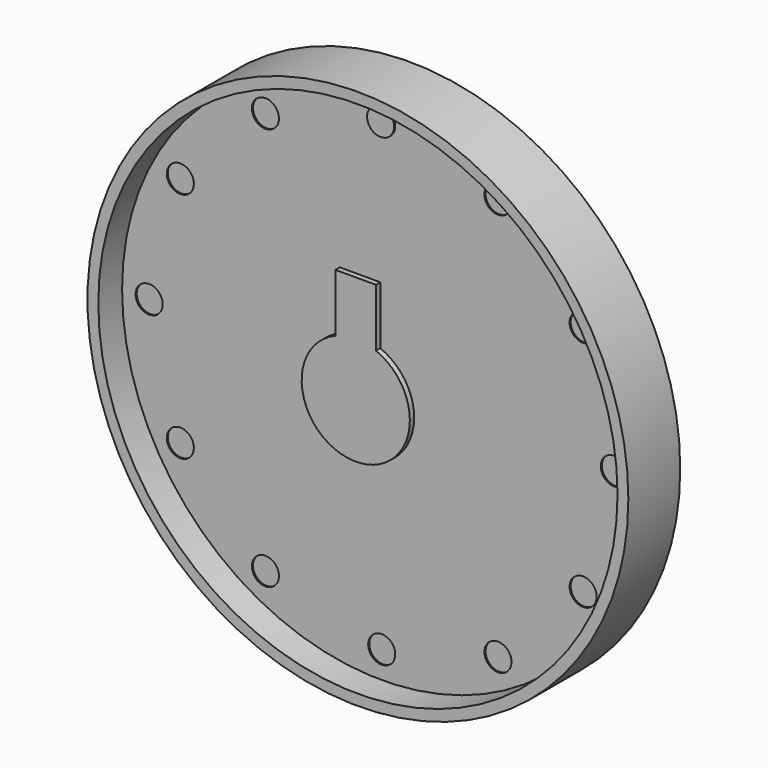
from build123d import *

# Parameters (mm, degrees)
F0_R      = 100
F1_DEPTH  = 24
F2_T      = -4
F3_R      = 5
F3_R_2    = 3
F4_DEPTH  = 6
F5_DEPTH  = 19
F6_DEPTH  = 8
F8_DEPTH  = 4
F10_DEPTH = 4
F11_R     = 5
F11_R_2   = 3
F12_DEPTH = 2
F13_R     = 98
F13_R_2   = 5
F14_DEPTH = 1
F16_R     = 5
F16_R_2   = 3
F17_DEPTH = 2
F18_R     = 5
F19_DEPTH = 0.5
F20_DEPTH = 1
F22_DEPTH = 2


with BuildPart() as f1:
    # F0 (on Front) → F1 (new body)
    with BuildSketch(Plane.XZ):
        Circle(F0_R)
    extrude(amount=F1_DEPTH)

    # F2
    f2_openings = [f1.faces().sort_by_distance(p)[0] for p in [
        (0, -24, 0),
    ]]
    offset(amount=F2_T, openings=f2_openings)

    # F3 (on Front) → F4 (join)
    with BuildSketch(Plane.XZ):
        with Locations((40, 0)):
            Circle(F3_R)
        with Locations((40, 0)):
            Circle(F3_R_2, mode=Mode.SUBTRACT)
        Circle(F3_R)
        Circle(F3_R_2, mode=Mode.SUBTRACT)
    extrude(amount=F4_DEPTH)


with BuildPart() as f5:
    # F5 (new): a face of the model
    f5_faces = [f1.part.faces().sort_by_distance(p)[0] for p in [
        (0, -4, 0),
    ]]
    extrude(f5_faces, amount=F5_DEPTH)

    # F7 (on face) → F8 (join)
    with BuildSketch(Plane.XZ.offset(6)):
        with BuildLine():
            ThreePointArc((9.2729637667, -1.3794085621), (9.3494561423, -0.6915886375), (9.375, 0))
            ThreePointArc((9.375, 0), (9.3494561423, 0.6915886375), (9.2729637667, 1.3794085621))
            ThreePointArc((9.2729637667, 1.3794085621), (8.9161548403, 2.8970343223), (8.3127812852, 4.3345463782))
            ThreePointArc((8.3127812852, 4.3345463782), (7.5845343223, 5.5104867402), (6.6911892658, 6.566476316))
            ThreePointArc((6.6911892658, 6.566476316), (5.5104867402, 7.5845343223), (4.1773988938, 8.3928519278))
            ThreePointArc((4.1773988938, 8.3928519278), (2.8970343223, 8.9161548403), (1.5536078905, 9.2453733036))
            ThreePointArc((1.5536078905, 9.2453733036), (0, 9.375), (-1.5536078905, 9.2453733036))
            ThreePointArc((-1.5536078905, 9.2453733036), (-2.8970343223, 8.9161548403), (-4.1773988938, 8.3928519278))
            ThreePointArc((-4.1773988938, 8.3928519278), (-5.5104867402, 7.5845343223), (-6.6911892658, 6.566476316))
            ThreePointArc((-6.6911892658, 6.566476316), (-7.5845343223, 5.5104867402), (-8.3127812852, 4.3345463782))
            ThreePointArc((-8.3127812852, 4.3345463782), (-8.9161548403, 2.8970343223), (-9.2729637667, 1.3794085621))
            ThreePointArc((-9.2729637667, 1.3794085621), (-9.375, 0), (-9.2729637667, -1.3794085621))
            ThreePointArc((-9.2729637667, -1.3794085621), (-8.9161548403, -2.8970343223), (-8.3127812852, -4.3345463782))
            ThreePointArc((-8.3127812852, -4.3345463782), (-7.5845343223, -5.5104867402), (-6.6911892658, -6.566476316))
            ThreePointArc((-6.6911892658, -6.566476316), (-5.5104867402, -7.5845343223), (-4.1773988938, -8.3928519278))
            ThreePointArc((-4.1773988938, -8.3928519278), (-2.8970343223, -8.9161548403), (-1.5536078905, -9.2453733036))
            ThreePointArc((-1.5536078905, -9.2453733036), (0, -9.375), (1.5536078905, -9.2453733036))
            ThreePointArc((1.5536078905, -9.2453733036), (2.8970343223, -8.9161548403), (4.1773988938, -8.3928519278))
            ThreePointArc((4.1773988938, -8.3928519278), (5.5104867402, -7.5845343223), (6.6911892658, -6.566476316))
            ThreePointArc((6.6911892658, -6.566476316), (7.5845343223, -5.5104867402), (8.3127812852, -4.3345463782))
            ThreePointArc((8.3127812852, -4.3345463782), (8.9161548403, -2.8970343223), (9.2729637667, -1.3794085621))
        make_face()
        with BuildLine():
            ThreePointArc((8.3127812852, 4.3345463782), (8.9161548403, 2.8970343223), (9.2729637667, 1.3794085621))
            Line((9.2729637667, 1.3794085621), (11.1823199426, 2.3946312492))
            Line((11.1823199426, 2.3946312492), (10.8182678729, 3.515068311))
            Line((10.8182678729, 3.515068311), (10.4542158031, 4.6355053728))
            Line((10.4542158031, 4.6355053728), (8.3127812852, 4.3345463782))
        make_face()
        with BuildLine():
            Line((11.1823199426, -2.3946312492), (9.2729637667, -1.3794085621))
            ThreePointArc((9.2729637667, -1.3794085621), (8.9161548403, -2.8970343223), (8.3127812852, -4.3345463782))
            Line((8.3127812852, -4.3345463782), (10.4542158031, -4.6355053728))
            Line((10.4542158031, -4.6355053728), (10.8182678729, -3.515068311))
            Line((10.8182678729, -3.515068311), (11.1823199426, -2.3946312492))
        make_face()
        with BuildLine():
            ThreePointArc((4.1773988938, 8.3928519278), (5.5104867402, 7.5845343223), (6.6911892658, 6.566476316))
            Line((6.6911892658, 6.566476316), (7.6391579371, 8.5101001246))
            Line((7.6391579371, 8.5101001246), (6.6860572448, 9.202568311))
            Line((6.6860572448, 9.202568311), (5.7329565525, 9.8950364974))
            Line((5.7329565525, 9.8950364974), (4.1773988938, 8.3928519278))
        make_face()
        with BuildLine():
            Line((7.6391579371, -8.5101001246), (6.6911892658, -6.566476316))
            ThreePointArc((6.6911892658, -6.566476316), (5.5104867402, -7.5845343223), (4.1773988938, -8.3928519278))
            Line((4.1773988938, -8.3928519278), (5.7329565525, -9.8950364974))
            Line((5.7329565525, -9.8950364974), (6.6860572448, -9.202568311))
            Line((6.6860572448, -9.202568311), (7.6391579371, -8.5101001246))
        make_face()
        with BuildLine():
            ThreePointArc((-1.5536078905, 9.2453733036), (0, 9.375), (1.5536078905, 9.2453733036))
            Line((1.5536078905, 9.2453733036), (1.1780972451, 11.375))
            Line((1.1780972451, 11.375), (0, 11.375))
            Line((0, 11.375), (-1.1780972451, 11.375))
            Line((-1.1780972451, 11.375), (-1.5536078905, 9.2453733036))
        make_face()
        with BuildLine():
            Line((1.1780972451, -11.375), (1.5536078905, -9.2453733036))
            ThreePointArc((1.5536078905, -9.2453733036), (0, -9.375), (-1.5536078905, -9.2453733036))
            Line((-1.5536078905, -9.2453733036), (-1.1780972451, -11.375))
            Line((-1.1780972451, -11.375), (0, -11.375))
            Line((0, -11.375), (1.1780972451, -11.375))
        make_face()
        with BuildLine():
            ThreePointArc((-6.6911892658, 6.566476316), (-5.5104867402, 7.5845343223), (-4.1773988938, 8.3928519278))
            Line((-4.1773988938, 8.3928519278), (-5.7329565525, 9.8950364974))
            Line((-5.7329565525, 9.8950364974), (-6.6860572448, 9.202568311))
            Line((-6.6860572448, 9.202568311), (-7.6391579371, 8.5101001246))
            Line((-7.6391579371, 8.5101001246), (-6.6911892658, 6.566476316))
        make_face()
        with BuildLine():
            Line((-5.7329565525, -9.8950364974), (-4.1773988938, -8.3928519278))
            ThreePointArc((-4.1773988938, -8.3928519278), (-5.5104867402, -7.5845343223), (-6.6911892658, -6.566476316))
            Line((-6.6911892658, -6.566476316), (-7.6391579371, -8.5101001246))
            Line((-7.6391579371, -8.5101001246), (-6.6860572448, -9.202568311))
            Line((-6.6860572448, -9.202568311), (-5.7329565525, -9.8950364974))
        make_face()
        with BuildLine():
            ThreePointArc((-9.2729637667, 1.3794085621), (-8.9161548403, 2.8970343223), (-8.3127812852, 4.3345463782))
            Line((-8.3127812852, 4.3345463782), (-10.4542158031, 4.6355053728))
            Line((-10.4542158031, 4.6355053728), (-10.8182678729, 3.515068311))
            Line((-10.8182678729, 3.515068311), (-11.1823199426, 2.3946312492))
            Line((-11.1823199426, 2.3946312492), (-9.2729637667, 1.3794085621))
        make_face()
        with BuildLine():
            Line((-10.4542158031, -4.6355053728), (-8.3127812852, -4.3345463782))
            ThreePointArc((-8.3127812852, -4.3345463782), (-8.9161548403, -2.8970343223), (-9.2729637667, -1.3794085621))
            Line((-9.2729637667, -1.3794085621), (-11.1823199426, -2.3946312492))
            Line((-11.1823199426, -2.3946312492), (-10.8182678729, -3.515068311))
            Line((-10.8182678729, -3.515068311), (-10.4542158031, -4.6355053728))
        make_face()
    extrude(amount=F8_DEPTH)

    # F21 (on face) → F22 (join)
    with BuildSketch(Plane.XZ.offset(23)):
        with BuildLine():
            ThreePointArc((-7.5, 18.5404962177), (-11.1803398875, -16.5831239518), (20, 0))
            ThreePointArc((20, 0), (16.5831239518, 11.1803398875), (7.5, 18.5404962177))
            ThreePointArc((7.5, 18.5404962177), (0, 20), (-7.5, 18.5404962177))
        make_face()
        with BuildLine():
            ThreePointArc((-7.5, 18.5404962177), (0, 20), (7.5, 18.5404962177))
            Line((7.5, 18.5404962177), (7.5, 40))
            Line((7.5, 40), (0, 40))
            Line((0, 40), (-7.5, 40))
            Line((-7.5, 40), (-7.5, 18.5404962177))
        make_face()
    extrude(amount=F22_DEPTH)


with BuildPart() as f6:
    # F6 (new): a face of the model
    f6_faces = [f1.part.faces().sort_by_distance(p)[0] for p in [
        (40, -4, 0),
    ]]
    extrude(f6_faces, amount=F6_DEPTH)

    # F9 (on face) → F10 (join)
    with BuildSketch(Plane.XZ.offset(6)):
        with BuildLine():
            ThreePointArc((68.0829066802, -1.5381733945), (68.1144747006, -0.7693746225), (68.125, 0))
            ThreePointArc((68.125, 0), (68.1144747006, 0.7693746225), (68.0829066802, 1.5381733945))
            ThreePointArc((68.0829066802, 1.5381733945), (67.9709283072, 2.9398630294), (67.7890320221, 4.3342039956))
            ThreePointArc((67.7890320221, 4.3342039956), (67.5104012706, 5.8475163042), (67.1494235596, 7.3433252263))
            ThreePointArc((67.1494235596, 7.3433252263), (66.7484645208, 8.6911029668), (66.280643318, 10.0171558733))
            ThreePointArc((66.280643318, 10.0171558733), (65.6934659962, 11.4394680865), (65.0293803521, 12.8275385085))
            ThreePointArc((65.0293803521, 12.8275385085), (64.3569644814, 14.0625), (63.6236643925, 15.2623099717))
            ThreePointArc((63.6236643925, 15.2623099717), (62.7536029668, 16.5314602207), (61.815433119, 17.7511268046))
            ThreePointArc((61.815433119, 17.7511268046), (60.9009482166, 18.8192983038), (59.934217974, 19.8404278876))
            ThreePointArc((59.934217974, 19.8404278876), (58.8192983038, 20.9009482166), (57.6480467764, 21.8989056799))
            ThreePointArc((57.6480467764, 21.8989056799), (56.5314602207, 22.7536029668), (55.3735505752, 23.5514238999))
            ThreePointArc((55.3735505752, 23.5514238999), (54.0625, 24.3569644814), (52.709356105, 25.0895972944))
            ThreePointArc((52.709356105, 25.0895972944), (51.4394680865, 25.6934659962), (50.1409852457, 26.2331096755))
            ThreePointArc((50.1409852457, 26.2331096755), (48.6911029668, 26.7484645208), (47.2152055856, 27.1837531139))
            ThreePointArc((47.2152055856, 27.1837531139), (45.8475163042, 27.5104012706), (44.4652101991, 27.7682826779))
            ThreePointArc((44.4652101991, 27.7682826779), (42.9398630294, 27.9709283072), (41.4057159597, 28.0898484802))
            ThreePointArc((41.4057159597, 28.0898484802), (40, 28.125), (38.5942840403, 28.0898484802))
            ThreePointArc((38.5942840403, 28.0898484802), (37.0601369706, 27.9709283072), (35.5347898009, 27.7682826779))
            ThreePointArc((35.5347898009, 27.7682826779), (34.1524836958, 27.5104012706), (32.7847944144, 27.1837531139))
            ThreePointArc((32.7847944144, 27.1837531139), (31.3088970332, 26.7484645208), (29.8590147543, 26.2331096755))
            ThreePointArc((29.8590147543, 26.2331096755), (28.5605319135, 25.6934659962), (27.290643895, 25.0895972944))
            ThreePointArc((27.290643895, 25.0895972944), (25.9375, 24.3569644814), (24.6264494248, 23.5514238999))
            ThreePointArc((24.6264494248, 23.5514238999), (23.4685397793, 22.7536029668), (22.3519532236, 21.8989056799))
            ThreePointArc((22.3519532236, 21.8989056799), (21.1807016962, 20.9009482166), (20.065782026, 19.8404278876))
            ThreePointArc((20.065782026, 19.8404278876), (19.0990517834, 18.8192983038), (18.184566881, 17.7511268046))
            ThreePointArc((18.184566881, 17.7511268046), (17.2463970332, 16.5314602207), (16.3763356075, 15.2623099717))
            ThreePointArc((16.3763356075, 15.2623099717), (15.6430355186, 14.0625), (14.9706196479, 12.8275385085))
            ThreePointArc((14.9706196479, 12.8275385085), (14.3065340038, 11.4394680865), (13.719356682, 10.0171558733))
            ThreePointArc((13.719356682, 10.0171558733), (13.2515354792, 8.6911029668), (12.8505764404, 7.3433252263))
            ThreePointArc((12.8505764404, 7.3433252263), (12.4895987294, 5.8475163042), (12.2109679779, 4.3342039956))
            ThreePointArc((12.2109679779, 4.3342039956), (12.0290716928, 2.9398630294), (11.9170933198, 1.5381733945))
            ThreePointArc((11.9170933198, 1.5381733945), (11.875, 0), (11.9170933198, -1.5381733945))
            ThreePointArc((11.9170933198, -1.5381733945), (12.0290716928, -2.9398630294), (12.2109679779, -4.3342039956))
            ThreePointArc((12.2109679779, -4.3342039956), (12.4895987294, -5.8475163042), (12.8505764404, -7.3433252263))
            ThreePointArc((12.8505764404, -7.3433252263), (13.2515354792, -8.6911029668), (13.719356682, -10.0171558733))
            ThreePointArc((13.719356682, -10.0171558733), (14.3065340038, -11.4394680865), (14.9706196479, -12.8275385085))
            ThreePointArc((14.9706196479, -12.8275385085), (15.6430355186, -14.0625), (16.3763356075, -15.2623099717))
            ThreePointArc((16.3763356075, -15.2623099717), (17.2463970332, -16.5314602207), (18.184566881, -17.7511268046))
            ThreePointArc((18.184566881, -17.7511268046), (19.0990517834, -18.8192983038), (20.065782026, -19.8404278876))
            ThreePointArc((20.065782026, -19.8404278876), (21.1807016962, -20.9009482166), (22.3519532236, -21.8989056799))
            ThreePointArc((22.3519532236, -21.8989056799), (23.4685397793, -22.7536029668), (24.6264494248, -23.5514238999))
            ThreePointArc((24.6264494248, -23.5514238999), (25.9375, -24.3569644814), (27.290643895, -25.0895972944))
            ThreePointArc((27.290643895, -25.0895972944), (28.5605319135, -25.6934659962), (29.8590147543, -26.2331096755))
            ThreePointArc((29.8590147543, -26.2331096755), (31.3088970332, -26.7484645208), (32.7847944144, -27.1837531139))
            ThreePointArc((32.7847944144, -27.1837531139), (34.1524836958, -27.5104012706), (35.5347898009, -27.7682826779))
            ThreePointArc((35.5347898009, -27.7682826779), (37.0601369706, -27.9709283072), (38.5942840403, -28.0898484802))
            ThreePointArc((38.5942840403, -28.0898484802), (40, -28.125), (41.4057159597, -28.0898484802))
            ThreePointArc((41.4057159597, -28.0898484802), (42.9398630294, -27.9709283072), (44.4652101991, -27.7682826779))
            ThreePointArc((44.4652101991, -27.7682826779), (45.8475163042, -27.5104012706), (47.2152055856, -27.1837531139))
            ThreePointArc((47.2152055856, -27.1837531139), (48.6911029668, -26.7484645208), (50.1409852457, -26.2331096755))
            ThreePointArc((50.1409852457, -26.2331096755), (51.4394680865, -25.6934659962), (52.709356105, -25.0895972944))
            ThreePointArc((52.709356105, -25.0895972944), (54.0625, -24.3569644814), (55.3735505752, -23.5514238999))
            ThreePointArc((55.3735505752, -23.5514238999), (56.5314602207, -22.7536029668), (57.6480467764, -21.8989056799))
            ThreePointArc((57.6480467764, -21.8989056799), (58.8192983038, -20.9009482166), (59.934217974, -19.8404278876))
            ThreePointArc((59.934217974, -19.8404278876), (60.9009482166, -18.8192983038), (61.815433119, -17.7511268046))
            ThreePointArc((61.815433119, -17.7511268046), (62.7536029668, -16.5314602207), (63.6236643925, -15.2623099717))
            ThreePointArc((63.6236643925, -15.2623099717), (64.3569644814, -14.0625), (65.0293803521, -12.8275385085))
            ThreePointArc((65.0293803521, -12.8275385085), (65.6934659962, -11.4394680865), (66.280643318, -10.0171558733))
            ThreePointArc((66.280643318, -10.0171558733), (66.7484645208, -8.6911029668), (67.1494235596, -7.3433252263))
            ThreePointArc((67.1494235596, -7.3433252263), (67.5104012706, -5.8475163042), (67.7890320221, -4.3342039956))
            ThreePointArc((67.7890320221, -4.3342039956), (67.9709283072, -2.9398630294), (68.0829066802, -1.5381733945))
        make_face()
        with BuildLine():
            ThreePointArc((68.0829066802, 1.5381733945), (68.1144747006, 0.7693746225), (68.125, 0))
            ThreePointArc((68.125, 0), (68.1144747006, -0.7693746225), (68.0829066802, -1.5381733945))
            Line((68.0829066802, -1.5381733945), (70.125, -1.1780972451))
            Line((70.125, -1.1780972451), (70.125, 0))
            Line((70.125, 0), (70.125, 1.1780972451))
            Line((70.125, 1.1780972451), (68.0829066802, 1.5381733945))
        make_face()
        with BuildLine():
            ThreePointArc((67.1494235596, 7.3433252263), (67.5104012706, 5.8475163042), (67.7890320221, 4.3342039956))
            Line((67.7890320221, 4.3342039956), (69.7116366623, 5.1109866922))
            Line((69.7116366623, 5.1109866922), (69.4666964721, 6.2633396859))
            Line((69.4666964721, 6.2633396859), (69.2217562819, 7.4156926796))
            Line((69.2217562819, 7.4156926796), (67.1494235596, 7.3433252263))
        make_face()
        with BuildLine():
            Line((69.7116366623, -5.1109866922), (67.7890320221, -4.3342039956))
            ThreePointArc((67.7890320221, -4.3342039956), (67.5104012706, -5.8475163042), (67.1494235596, -7.3433252263))
            Line((67.1494235596, -7.3433252263), (69.2217562819, -7.4156926796))
            Line((69.2217562819, -7.4156926796), (69.4666964721, -6.2633396859))
            Line((69.4666964721, -6.2633396859), (69.7116366623, -5.1109866922))
        make_face()
        with BuildLine():
            ThreePointArc((65.0293803521, 12.8275385085), (65.6934659962, 11.4394680865), (66.280643318, 10.0171558733))
            Line((66.280643318, 10.0171558733), (67.9997322302, 11.1766959857))
            Line((67.9997322302, 11.1766959857), (67.5205569115, 12.2529413727))
            Line((67.5205569115, 12.2529413727), (67.0413815928, 13.3291867596))
            Line((67.0413815928, 13.3291867596), (65.0293803521, 12.8275385085))
        make_face()
        with BuildLine():
            Line((67.9997322302, -11.1766959857), (66.280643318, -10.0171558733))
            ThreePointArc((66.280643318, -10.0171558733), (65.6934659962, -11.4394680865), (65.0293803521, -12.8275385085))
            Line((65.0293803521, -12.8275385085), (67.0413815928, -13.3291867596))
            Line((67.0413815928, -13.3291867596), (67.5205569115, -12.2529413727))
            Line((67.5205569115, -12.2529413727), (67.9997322302, -11.1766959857))
        make_face()
        with BuildLine():
            ThreePointArc((61.815433119, 17.7511268046), (62.7536029668, 16.5314602207), (63.6236643925, 15.2623099717))
            Line((63.6236643925, 15.2623099717), (65.064105142, 16.753930033))
            Line((65.064105142, 16.753930033), (64.3716369555, 17.7070307253))
            Line((64.3716369555, 17.7070307253), (63.6791687691, 18.6601314176))
            Line((63.6791687691, 18.6601314176), (61.815433119, 17.7511268046))
        make_face()
        with BuildLine():
            Line((65.064105142, -16.753930033), (63.6236643925, -15.2623099717))
            ThreePointArc((63.6236643925, -15.2623099717), (62.7536029668, -16.5314602207), (61.815433119, -17.7511268046))
            Line((61.815433119, -17.7511268046), (63.6791687691, -18.6601314176))
            Line((63.6791687691, -18.6601314176), (64.3716369555, -17.7070307253))
            Line((64.3716369555, -17.7070307253), (65.064105142, -16.753930033))
        make_face()
        with BuildLine():
            ThreePointArc((57.6480467764, 21.8989056799), (58.8192983038, 20.9009482166), (59.934217974, 19.8404278876))
            Line((59.934217974, 19.8404278876), (61.0330563882, 21.5989369435))
            Line((61.0330563882, 21.5989369435), (60.1575595166, 22.3872378675))
            Line((60.1575595166, 22.3872378675), (59.282062645, 23.1755387915))
            Line((59.282062645, 23.1755387915), (57.6480467764, 21.8989056799))
        make_face()
        with BuildLine():
            Line((61.0330563882, -21.5989369435), (59.934217974, -19.8404278876))
            ThreePointArc((59.934217974, -19.8404278876), (58.8192983038, -20.9009482166), (57.6480467764, -21.8989056799))
            Line((57.6480467764, -21.8989056799), (59.282062645, -23.1755387915))
            Line((59.282062645, -23.1755387915), (60.1575595166, -22.3872378675))
            Line((60.1575595166, -22.3872378675), (61.0330563882, -21.5989369435))
        make_face()
        with BuildLine():
            ThreePointArc((52.709356105, 25.0895972944), (54.0625, 24.3569644814), (55.3735505752, 23.5514238999))
            Line((55.3735505752, 23.5514238999), (56.0827621424, 25.4999666665))
            Line((56.0827621424, 25.4999666665), (55.0625, 26.089015289))
            Line((55.0625, 26.089015289), (54.0422378576, 26.6780639116))
            Line((54.0422378576, 26.6780639116), (52.709356105, 25.0895972944))
        make_face()
        with BuildLine():
            Line((56.0827621424, -25.4999666665), (55.3735505752, -23.5514238999))
            ThreePointArc((55.3735505752, -23.5514238999), (54.0625, -24.3569644814), (52.709356105, -25.0895972944))
            Line((52.709356105, -25.0895972944), (54.0422378576, -26.6780639116))
            Line((54.0422378576, -26.6780639116), (55.0625, -26.089015289))
            Line((55.0625, -26.089015289), (56.0827621424, -25.4999666665))
        make_face()
        with BuildLine():
            ThreePointArc((47.2152055856, 27.1837531139), (48.6911029668, 26.7484645208), (50.1409852457, 26.2331096755))
            Line((50.1409852457, 26.2331096755), (50.4295740173, 28.2865254836))
            Line((50.4295740173, 28.2865254836), (49.3091369555, 28.6505775534))
            Line((49.3091369555, 28.6505775534), (48.1886998938, 29.0146296232))
            Line((48.1886998938, 29.0146296232), (47.2152055856, 27.1837531139))
        make_face()
        with BuildLine():
            Line((50.4295740173, -28.2865254836), (50.1409852457, -26.2331096755))
            ThreePointArc((50.1409852457, -26.2331096755), (48.6911029668, -26.7484645208), (47.2152055856, -27.1837531139))
            Line((47.2152055856, -27.1837531139), (48.1886998938, -29.0146296232))
            Line((48.1886998938, -29.0146296232), (49.3091369555, -28.6505775534))
            Line((49.3091369555, -28.6505775534), (50.4295740173, -28.2865254836))
        make_face()
        with BuildLine():
            ThreePointArc((41.4057159597, 28.0898484802), (42.9398630294, 27.9709283072), (44.4652101991, 27.7682826779))
            Line((44.4652101991, 27.7682826779), (44.3205634611, 29.8368274034))
            Line((44.3205634611, 29.8368274034), (43.1489199559, 29.959972098))
            Line((43.1489199559, 29.959972098), (41.9772764508, 30.0831167926))
            Line((41.9772764508, 30.0831167926), (41.4057159597, 28.0898484802))
        make_face()
        with BuildLine():
            Line((44.3205634611, -29.8368274034), (44.4652101991, -27.7682826779))
            ThreePointArc((44.4652101991, -27.7682826779), (42.9398630294, -27.9709283072), (41.4057159597, -28.0898484802))
            Line((41.4057159597, -28.0898484802), (41.9772764508, -30.0831167926))
            Line((41.9772764508, -30.0831167926), (43.1489199559, -29.959972098))
            Line((43.1489199559, -29.959972098), (44.3205634611, -29.8368274034))
        make_face()
        with BuildLine():
            ThreePointArc((35.5347898009, 27.7682826779), (37.0601369706, 27.9709283072), (38.5942840403, 28.0898484802))
            Line((38.5942840403, 28.0898484802), (38.0227235492, 30.0831167926))
            Line((38.0227235492, 30.0831167926), (36.8510800441, 29.959972098))
            Line((36.8510800441, 29.959972098), (35.6794365389, 29.8368274034))
            Line((35.6794365389, 29.8368274034), (35.5347898009, 27.7682826779))
        make_face()
        with BuildLine():
            Line((38.0227235492, -30.0831167926), (38.5942840403, -28.0898484802))
            ThreePointArc((38.5942840403, -28.0898484802), (37.0601369706, -27.9709283072), (35.5347898009, -27.7682826779))
            Line((35.5347898009, -27.7682826779), (35.6794365389, -29.8368274034))
            Line((35.6794365389, -29.8368274034), (36.8510800441, -29.959972098))
            Line((36.8510800441, -29.959972098), (38.0227235492, -30.0831167926))
        make_face()
        with BuildLine():
            ThreePointArc((29.8590147543, 26.2331096755), (31.3088970332, 26.7484645208), (32.7847944144, 27.1837531139))
            Line((32.7847944144, 27.1837531139), (31.8113001062, 29.0146296232))
            Line((31.8113001062, 29.0146296232), (30.6908630445, 28.6505775534))
            Line((30.6908630445, 28.6505775534), (29.5704259827, 28.2865254836))
            Line((29.5704259827, 28.2865254836), (29.8590147543, 26.2331096755))
        make_face()
        with BuildLine():
            Line((31.8113001062, -29.0146296232), (32.7847944144, -27.1837531139))
            ThreePointArc((32.7847944144, -27.1837531139), (31.3088970332, -26.7484645208), (29.8590147543, -26.2331096755))
            Line((29.8590147543, -26.2331096755), (29.5704259827, -28.2865254836))
            Line((29.5704259827, -28.2865254836), (30.6908630445, -28.6505775534))
            Line((30.6908630445, -28.6505775534), (31.8113001062, -29.0146296232))
        make_face()
        with BuildLine():
            ThreePointArc((24.6264494248, 23.5514238999), (25.9375, 24.3569644814), (27.290643895, 25.0895972944))
            Line((27.290643895, 25.0895972944), (25.9577621424, 26.6780639116))
            Line((25.9577621424, 26.6780639116), (24.9375, 26.089015289))
            Line((24.9375, 26.089015289), (23.9172378576, 25.4999666665))
            Line((23.9172378576, 25.4999666665), (24.6264494248, 23.5514238999))
        make_face()
        with BuildLine():
            Line((25.9577621424, -26.6780639116), (27.290643895, -25.0895972944))
            ThreePointArc((27.290643895, -25.0895972944), (25.9375, -24.3569644814), (24.6264494248, -23.5514238999))
            Line((24.6264494248, -23.5514238999), (23.9172378576, -25.4999666665))
            Line((23.9172378576, -25.4999666665), (24.9375, -26.089015289))
            Line((24.9375, -26.089015289), (25.9577621424, -26.6780639116))
        make_face()
        with BuildLine():
            ThreePointArc((20.065782026, 19.8404278876), (21.1807016962, 20.9009482166), (22.3519532236, 21.8989056799))
            Line((22.3519532236, 21.8989056799), (20.717937355, 23.1755387915))
            Line((20.717937355, 23.1755387915), (19.8424404834, 22.3872378675))
            Line((19.8424404834, 22.3872378675), (18.9669436118, 21.5989369435))
            Line((18.9669436118, 21.5989369435), (20.065782026, 19.8404278876))
        make_face()
        with BuildLine():
            Line((20.717937355, -23.1755387915), (22.3519532236, -21.8989056799))
            ThreePointArc((22.3519532236, -21.8989056799), (21.1807016962, -20.9009482166), (20.065782026, -19.8404278876))
            Line((20.065782026, -19.8404278876), (18.9669436118, -21.5989369435))
            Line((18.9669436118, -21.5989369435), (19.8424404834, -22.3872378675))
            Line((19.8424404834, -22.3872378675), (20.717937355, -23.1755387915))
        make_face()
        with BuildLine():
            ThreePointArc((16.3763356075, 15.2623099717), (17.2463970332, 16.5314602207), (18.184566881, 17.7511268046))
            Line((18.184566881, 17.7511268046), (16.3208312309, 18.6601314176))
            Line((16.3208312309, 18.6601314176), (15.6283630445, 17.7070307253))
            Line((15.6283630445, 17.7070307253), (14.935894858, 16.753930033))
            Line((14.935894858, 16.753930033), (16.3763356075, 15.2623099717))
        make_face()
        with BuildLine():
            Line((16.3208312309, -18.6601314176), (18.184566881, -17.7511268046))
            ThreePointArc((18.184566881, -17.7511268046), (17.2463970332, -16.5314602207), (16.3763356075, -15.2623099717))
            Line((16.3763356075, -15.2623099717), (14.935894858, -16.753930033))
            Line((14.935894858, -16.753930033), (15.6283630445, -17.7070307253))
            Line((15.6283630445, -17.7070307253), (16.3208312309, -18.6601314176))
        make_face()
        with BuildLine():
            ThreePointArc((13.719356682, 10.0171558733), (14.3065340038, 11.4394680865), (14.9706196479, 12.8275385085))
            Line((14.9706196479, 12.8275385085), (12.9586184072, 13.3291867596))
            Line((12.9586184072, 13.3291867596), (12.4794430885, 12.2529413727))
            Line((12.4794430885, 12.2529413727), (12.0002677698, 11.1766959857))
            Line((12.0002677698, 11.1766959857), (13.719356682, 10.0171558733))
        make_face()
        with BuildLine():
            Line((12.9586184072, -13.3291867596), (14.9706196479, -12.8275385085))
            ThreePointArc((14.9706196479, -12.8275385085), (14.3065340038, -11.4394680865), (13.719356682, -10.0171558733))
            Line((13.719356682, -10.0171558733), (12.0002677698, -11.1766959857))
            Line((12.0002677698, -11.1766959857), (12.4794430885, -12.2529413727))
            Line((12.4794430885, -12.2529413727), (12.9586184072, -13.3291867596))
        make_face()
        with BuildLine():
            ThreePointArc((12.2109679779, 4.3342039956), (12.4895987294, 5.8475163042), (12.8505764404, 7.3433252263))
            Line((12.8505764404, 7.3433252263), (10.7782437181, 7.4156926796))
            Line((10.7782437181, 7.4156926796), (10.5333035279, 6.2633396859))
            Line((10.5333035279, 6.2633396859), (10.2883633377, 5.1109866922))
            Line((10.2883633377, 5.1109866922), (12.2109679779, 4.3342039956))
        make_face()
        with BuildLine():
            Line((10.7782437181, -7.4156926796), (12.8505764404, -7.3433252263))
            ThreePointArc((12.8505764404, -7.3433252263), (12.4895987294, -5.8475163042), (12.2109679779, -4.3342039956))
            Line((12.2109679779, -4.3342039956), (10.2883633377, -5.1109866922))
            Line((10.2883633377, -5.1109866922), (10.5333035279, -6.2633396859))
            Line((10.5333035279, -6.2633396859), (10.7782437181, -7.4156926796))
        make_face()
        with BuildLine():
            ThreePointArc((11.9170933198, -1.5381733945), (11.875, 0), (11.9170933198, 1.5381733945))
            Line((11.9170933198, 1.5381733945), (9.875, 1.1780972451))
            Line((9.875, 1.1780972451), (9.875, 0))
            Line((9.875, 0), (9.875, -1.1780972451))
            Line((9.875, -1.1780972451), (11.9170933198, -1.5381733945))
        make_face()
    extrude(amount=F10_DEPTH)


with BuildPart() as f12:
    # F11 (on face) → F12 (new body)
    with BuildSketch(Plane.XZ.offset(10)):
        Circle(F11_R)
        Circle(F11_R_2, mode=Mode.SUBTRACT)
    extrude(amount=F12_DEPTH)


with BuildPart() as f14:
    # F13 (on face) → F14 (new body)
    with BuildSketch(Plane.XZ.offset(12)):
        Circle(F13_R)
        Circle(F13_R_2, mode=Mode.SUBTRACT)
    extrude(amount=F14_DEPTH)


with BuildPart() as f1_1:
    add(f1.part)

    # F15: cut F14
    add(f14.part, mode=Mode.SUBTRACT)


with BuildPart() as f17:
    # F16 (on face) → F17 (new body, through all)
    with BuildSketch(Plane(origin=(0, -12, 0), x_dir=(-1, 0, 0), z_dir=(0, 1, 0))):
        with Locations((-40, 0)):
            Circle(F16_R)
        with Locations((-40, 0)):
            Circle(F16_R_2, mode=Mode.SUBTRACT)
    extrude(amount=F17_DEPTH)


with BuildPart() as f14_1:
    add(f14.part)

    # F18 (on face) → F19 (cut)
    with BuildSketch(Plane.XZ.offset(13)):
        with Locations((0, 86)):
            Circle(F18_R)
        with Locations((-43, 74.4781847255)):
            Circle(F18_R)
        with Locations((-74.4781847255, 43)):
            Circle(F18_R)
        with Locations((-86, 0)):
            Circle(F18_R)
        with Locations((-74.4781847255, -43)):
            Circle(F18_R)
        with Locations((-43, -74.4781847255)):
            Circle(F18_R)
        with Locations((0, -86)):
            Circle(F18_R)
        with Locations((43, -74.4781847255)):
            Circle(F18_R)
        with Locations((74.4781847255, -43)):
            Circle(F18_R)
        with Locations((86, 0)):
            Circle(F18_R)
        with Locations((74.4781847255, 43)):
            Circle(F18_R)
        with Locations((43, 74.4781847255)):
            Circle(F18_R)
    extrude(amount=-F19_DEPTH, mode=Mode.SUBTRACT)


with BuildPart() as f20:
    # F20 (new): a face of the model
    f20_faces = [f14_1.part.faces().sort_by_distance(p)[0] for p in [
        (0, -12.5, 86),
    ]]
    extrude(f20_faces, amount=F20_DEPTH)


solid = Compound([f5.part, f6.part, f12.part, f1_1.part, f17.part, f14_1.part, f20.part])
